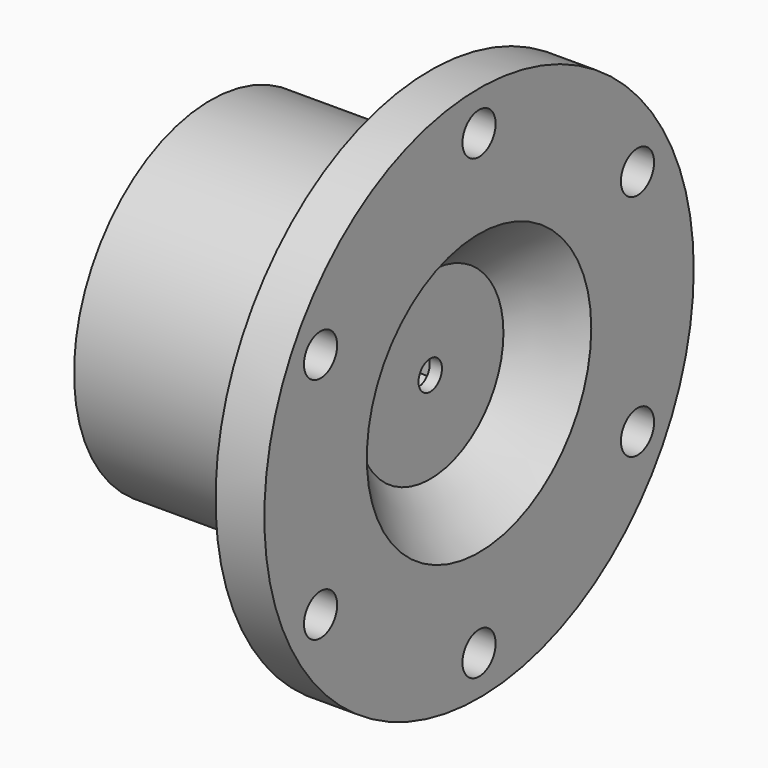
from build123d import *

# Parameters (mm, degrees)
F0_R      = 17.78
F0_R_2    = 15.24
F1_DEPTH  = 17.78
F2_R      = 17.78
F3_DEPTH  = 5.08
F4_R      = 1.524
F5_DEPTH  = 25.4
F6_R      = 27.94
F6_R_2    = 2.159
F6_R_3    = 9.525
F7_DEPTH  = 5.08
F8_SIZE   = 5.07999
F10_DEPTH = 3.81


# Not quite as in the source:
# - a fillet or chamfer is up to 0.001 mm smaller than in the source, because OpenCascade refuses the exact size


with BuildPart() as f1:
    # F0 (on Right) → F1 (new body)
    with BuildSketch(Plane.YZ):
        Circle(F0_R)
        Circle(F0_R_2, mode=Mode.SUBTRACT)
    extrude(amount=F1_DEPTH)

    # F2 (on face) → F3 (join)
    with BuildSketch(Plane.YZ.offset(17.78)):
        Circle(F2_R)
    extrude(amount=F3_DEPTH)

    # F4 (on face) → F5 (cut)
    with BuildSketch(Plane.YZ.offset(22.86)):
        Circle(F4_R)
    extrude(amount=-F5_DEPTH, mode=Mode.SUBTRACT)

    # F6 (on face) → F7 (join)
    with BuildSketch(Plane.YZ.offset(22.86)):
        Circle(F6_R)
        with Locations((0, -23.8125)):
            Circle(F6_R_2, mode=Mode.SUBTRACT)
        with Locations((-20.6222299276, -11.90625)):
            Circle(F6_R_2, mode=Mode.SUBTRACT)
        Circle(F6_R_3, mode=Mode.SUBTRACT)
        with Locations((20.6222299276, -11.90625)):
            Circle(F6_R_2, mode=Mode.SUBTRACT)
        with Locations((-20.6222299276, 11.90625)):
            Circle(F6_R_2, mode=Mode.SUBTRACT)
        with Locations((0, 23.8125)):
            Circle(F6_R_2, mode=Mode.SUBTRACT)
        with Locations((20.6222299276, 11.90625)):
            Circle(F6_R_2, mode=Mode.SUBTRACT)
    extrude(amount=F7_DEPTH)

    # F8 (size 5.08 in the source; OpenCascade refuses exactly that, so slightly less here)
    f8_edges = [f1.edges().sort_by_distance(p)[0] for p in [
        (27.94, -9.525, 0),
    ]]
    chamfer(f8_edges, length=F8_SIZE)

    # F9 (on face) → F10 (cut)
    with BuildSketch(Plane(origin=(17.78, 0, 0), x_dir=(0, -1, 0), z_dir=(-1, 0, 0))):
        with BuildLine():
            ThreePointArc((3.3655, 2.413), (0, 4.437080139), (-3.3655, 2.413))
            Line((-3.3655, 2.413), (-3.3655, -2.413))
            ThreePointArc((-3.3655, -2.413), (0, -4.437080139), (3.3655, -2.413))
            Line((3.3655, -2.413), (3.3655, 2.413))
        make_face()
    extrude(amount=-F10_DEPTH, mode=Mode.SUBTRACT)


solid = f1.part
